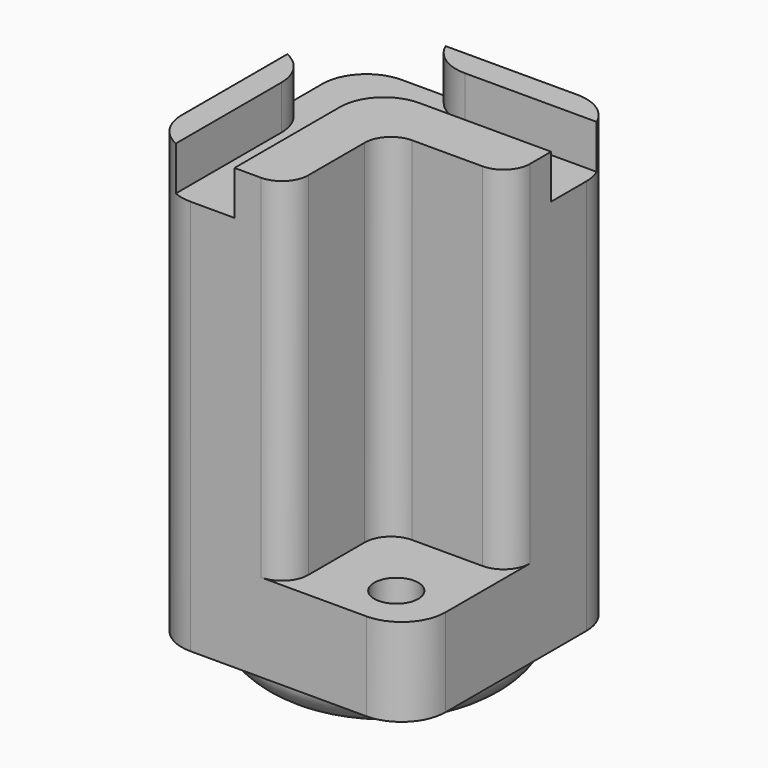
from build123d import *

# Parameters (mm, degrees)
F0_W         = 30
F0_H         = 30
F1_DEPTH     = 10
F3_DEPTH     = 40
F4_W         = 7
F4_H         = 3
F4_W_2       = 3
F4_H_2       = 7
F4_H_3       = 20
F4_W_3       = 20
F5_DEPTH     = 5
F6_R         = 2.5
F7_DEPTH     = 10
F10_R        = 5
F11_T1_DEPTH = 17.5
F11_T3_DEPTH = 16.4564392374
F12_R        = 3


# Not quite as in the source:
# - a fillet or chamfer that OpenCascade refuses, or shapes differently, is made with other operations: its cross-section is extruded or revolved along the edge and cut away or added


with BuildPart() as f1:
    # F0 (on Top) → F1 (new body)
    with BuildSketch(Plane.XY):
        Rectangle(F0_W, F0_H)
    extrude(amount=F1_DEPTH)

    # F2 (on face) → F3 (join)
    with BuildSketch(Plane.XY.offset(10)):
        Polygon((15, 15), (-15, 15), (-15, -15), (1, -15), (1, -1), (15, -1), align=None)
    extrude(amount=F3_DEPTH)

    # F4 (on face) → F5 (cut)
    with BuildSketch(Plane.XY.offset(50)):
        with Locations((-8.5, 13.5)):
            Rectangle(F4_W, F4_H)
        with Locations((-13.5, 13.5)):
            Rectangle(F4_W_2, F4_H)
        with Locations((-8.5, 8.5)):
            Rectangle(F4_W, F4_H_2)
        with Locations((-13.5, 8.5)):
            Rectangle(F4_W_2, F4_H_2)
        with Locations((-8.5, -5)):
            Rectangle(F4_W, F4_H_3)
        with Locations((5, 8.5)):
            Rectangle(F4_W_3, F4_H_2)
    extrude(amount=-F5_DEPTH, mode=Mode.SUBTRACT)

    # F6 (on face) → F7 (cut, through all)
    with BuildSketch(Plane.XY.offset(10)):
        with Locations((9, -9.5)):
            Circle(F6_R)
    extrude(amount=-F7_DEPTH, mode=Mode.SUBTRACT)

    # F8 (on Front) → F9 (revolve)
    with BuildSketch(Plane.XZ):
        with BuildLine():
            Line((0, 0), (-14.5, 0))
            add(Edge.make_bspline(
                [(-14.5, 0), (-14.5131281167, -2.1023036255), (-8.5269566385, -5.7796890584), (-3.0055961106, -6.062279921), (0, -6.0380934738)],
                knots=[0, 0, 0, 0, 0.4748413397, 1, 1, 1, 1], degree=3))
            Line((0, -6.0380934738), (0, 0))
        make_face()
    revolve(axis=Axis((0, 0, -7.25), (0, 0, -1)))

    # F10
    f10_edges = [f1.edges().sort_by_distance(p)[0] for p in [
        (-15, -15, 25),
        (15, -15, 5),
        (-15, 15, 22.5),
        (15, 15, 25),
    ]]
    fillet(f10_edges, radius=F10_R)

    # F11: fillet of radius 5 on 3 edges, made by hand

    # F11_s2 → F11_t1 (cut)
    with BuildSketch(Plane.XY.offset(45)):
        with BuildLine():
            ThreePointArc((-5, 0), (-3.5355339059, 3.5355339059), (0, 5))
            Line((0, 5), (-5, 5))
            Line((-5, 5), (-5, 0))
        make_face()
    extrude(amount=F11_T1_DEPTH, mode=Mode.SUBTRACT)

    # F11_s4 → F11_t3 (cut)
    with BuildSketch(Plane.XY.offset(45)):
        with BuildLine():
            ThreePointArc((-5, 15), (-3.1560370926, 12.8166998673), (-0.417424305, 12))
            Line((-0.417424305, 12), (-5, 12))
            Line((-5, 12), (-5, 15))
        make_face()
        with BuildLine():
            ThreePointArc((-12, 0.417424305), (-12.8166998673, 3.1560370926), (-15, 5))
            Line((-15, 5), (-12, 5))
            Line((-12, 5), (-12, 0.417424305))
        make_face()
    extrude(amount=F11_T3_DEPTH, mode=Mode.SUBTRACT)

    # F12
    f12_edges = [f1.edges().sort_by_distance(p)[0] for p in [
        (1, -1, 30),
        (1, -15, 30),
        (15, -1, 30),
    ]]
    fillet(f12_edges, radius=F12_R)


solid = f1.part
